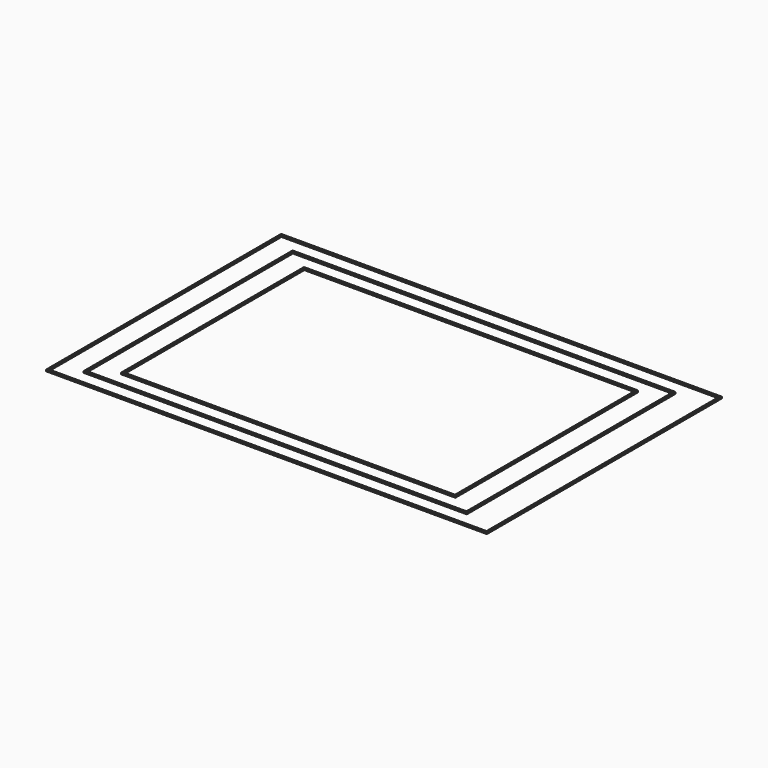
from build123d import *

# Parameters (mm, degrees)
F1_W     = 270
F1_H     = 180
F1_W_2   = 268
F1_H_2   = 178
F2_DEPTH = 1
F1_W_3   = 234.7133469
F1_H_3   = 160
F1_W_4   = 232.7133469
F1_H_4   = 158
F1_W_5   = 204.7133469
F1_H_5   = 140
F1_W_6   = 202.7133469
F1_H_6   = 138


# Not quite as in the source:
# - a feature names something its author has since deleted; it is built from what else it names


with BuildPart() as f2:
    # F1 (on Top) → F2 (new body)
    with BuildSketch(Plane.XY):
        with Locations((43.5175617039, 17.8632308638)):
            Rectangle(F1_W, F1_H)
        with Locations((43.5175617039, 17.8632308638)):
            Rectangle(F1_W_2, F1_H_2, mode=Mode.SUBTRACT)
    extrude(amount=F2_DEPTH)


with BuildPart() as f2b:
    # F1 (on Top) → F2, piece 2 (new body)
    with BuildSketch(Plane.XY):
        with Locations((40.8742351539, 17.8632308638)):
            Rectangle(F1_W_3, F1_H_3)
        with Locations((40.8742351539, 17.8632308638)):
            Rectangle(F1_W_4, F1_H_4, mode=Mode.SUBTRACT)
    extrude(amount=F2_DEPTH)


with BuildPart() as f2c:
    # F1 (on Top) → F2, piece 3 (new body)
    with BuildSketch(Plane.XY):
        with Locations((40.8742351539, 17.8632308638)):
            Rectangle(F1_W_5, F1_H_5)
        with Locations((40.8742351539, 17.8632308638)):
            Rectangle(F1_W_6, F1_H_6, mode=Mode.SUBTRACT)
    extrude(amount=F2_DEPTH)


solid = Compound([f2.part, f2b.part, f2c.part])
